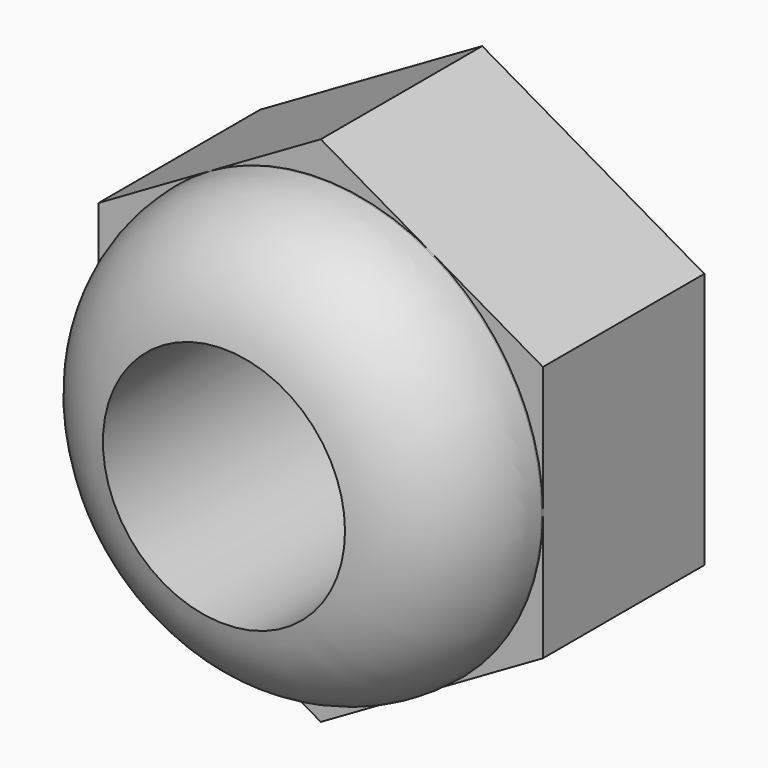
from build123d import *

# Parameters (mm, degrees)
F1_DEPTH = 2.5
F2_R     = 2.7521630024
F3_DEPTH = 1.5
F4_R     = 1.5
F5_DEPTH = 4


# Not quite as in the source:
# - a fillet or chamfer that OpenCascade refuses, or shapes differently, is made with other operations: its cross-section is extruded or revolved along the edge and cut away or added


with BuildPart() as f1:
    # F0 (on Front) → F1 (new body)
    with BuildSketch(Plane.XZ):
        Polygon((0, -3.1779241005), (2.7521630024, -1.5889620503), (2.7521630024, 1.5889620503), (0, 3.1779241005), (-2.7521630024, 1.5889620503), (-2.7521630024, -1.5889620503), align=None)
    extrude(amount=F1_DEPTH)

    # F2 (on face) → F3 (join)
    with BuildSketch(Plane.XZ.offset(2.5)):
        Circle(F2_R)
    extrude(amount=F3_DEPTH)

    # F4 (on face) → F5 (cut, through all)
    with BuildSketch(Plane.XZ.offset(4)):
        Circle(F4_R)
    extrude(amount=-F5_DEPTH, mode=Mode.SUBTRACT)

    # F6: fillet of radius 1.5 on 1 edges, made by hand

    # F6_s1 → F6_t2 (revolve, cut)
    with BuildSketch(Plane.XY):
        with BuildLine():
            ThreePointArc((2.7521630024, -2.5206160665), (2.3970986985, -3.4896992682), (1.5, -4))
            Line((1.5, -4), (2.7521630024, -4))
            Line((2.7521630024, -4), (2.7521630024, -2.5206160665))
        make_face()
    revolve(axis=Axis((0, -4, 0), (0, -1, 0)), mode=Mode.SUBTRACT)


solid = f1.part
